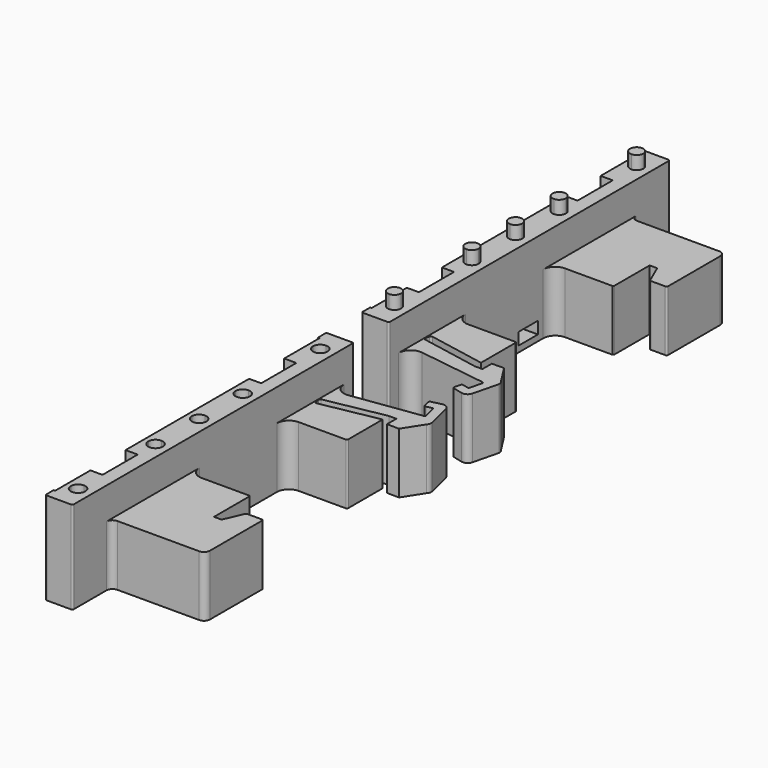
from build123d import *

# Parameters (mm, degrees)
F0_W      = 0.25
F0_H      = 7.25
F0_W_2    = 2
F0_H_2    = 25.5
F1_DEPTH  = 3.5
F2_W      = 4
F2_H      = 2
F3_DEPTH  = 4.5
F5_DEPTH  = 6.5
F7_DEPTH  = 5.25
F9_ANGLE  = 180
F13_DEPTH = 2.4
F14_DEPTH = 2.2


# Not quite as in the source:
# - a feature names something its author has since deleted; it is built from what else it names


with BuildPart() as f1:
    # F0 (on Top) → F1 (new body)
    with BuildSketch(Plane.XY):
        with BuildLine():
            Line((-24.9246123582, 55.1439750494), (-24.9246123582, 35.9745444804))
            ThreePointArc((-24.9246123582, 35.9745444804), (-24.3388259206, 37.3887580428), (-22.9246123582, 37.9745444804))
            Line((-22.9246123582, 37.9745444804), (-15.1132449657, 37.9745444804))
            ThreePointArc((-15.1132449657, 37.9745444804), (-14.974931029, 38.0663469276), (-14.9246123582, 38.2245444804))
            Line((-14.9246123582, 38.2245444804), (-14.9246123582, 45.4523755611))
            Line((-14.9246123582, 45.4523755611), (-13.6746123582, 45.4523755611))
            Line((-13.6746123582, 45.4523755611), (-12.3013395786, 42.2942820054))
            ThreePointArc((-12.3013395786, 42.2942820054), (-12.2091477453, 42.1849017835), (-12.0720770719, 42.1439750494))
            Line((-12.0720770719, 42.1439750494), (-9.7359797508, 42.1439750494))
            ThreePointArc((-9.7359797508, 42.1439750494), (-9.5179749824, 42.1913560505), (-9.4246123582, 42.3939750494))
            Line((-9.4246123582, 42.3939750494), (-9.4246123582, 53.1439750494))
            ThreePointArc((-9.4246123582, 53.1439750494), (-9.717505577, 53.8510818306), (-10.4246123582, 54.1439750494))
            Line((-10.4246123582, 54.1439750494), (-23.9246123582, 54.1439750494))
            ThreePointArc((-23.9246123582, 54.1439750494), (-24.6317191394, 54.4368682682), (-24.9246123582, 55.1439750494))
        make_face()
        with Locations((-29.2996123582, 16.7689750494)):
            Rectangle(F0_W, F0_H)
        with Locations((-29.2996123582, 49.5189750494)):
            Rectangle(F0_W, F0_H)
        with Locations((-29.2996123582, 56.7689750494)):
            Rectangle(F0_W, F0_H)
        with BuildLine():
            Line((-29.4246123582, 5.8939750494), (-29.4246123582, 4.3939750494))
            ThreePointArc((-29.4246123582, 4.3939750494), (-29.3513890535, 4.2171983541), (-29.1746123582, 4.1439750494))
            Line((-29.1746123582, 4.1439750494), (-25.2605436295, 4.1439750494))
            ThreePointArc((-25.2605436295, 4.1439750494), (-25.0248826881, 4.1780111688), (-24.9246123582, 4.3939750494))
            Line((-24.9246123582, 4.3939750494), (-24.9246123582, 6.1439750494))
            Line((-24.9246123582, 6.1439750494), (-24.9246123582, 19.9745444804))
            Line((-24.9246123582, 19.9745444804), (-24.9246123582, 35.9745444804))
            Line((-24.9246123582, 35.9745444804), (-24.9246123582, 55.1439750494))
            Line((-24.9246123582, 55.1439750494), (-24.9246123582, 61.8939750494))
            ThreePointArc((-24.9246123582, 61.8939750494), (-24.9978356629, 62.0707517447), (-25.1746123582, 62.1439750494))
            Line((-25.1746123582, 62.1439750494), (-29.1746123582, 62.1439750494))
            ThreePointArc((-29.1746123582, 62.1439750494), (-29.3513890535, 62.0707517447), (-29.4246123582, 61.8939750494))
            Line((-29.4246123582, 61.8939750494), (-29.4246123582, 60.3939750494))
            Line((-29.4246123582, 60.3939750494), (-29.1746123582, 60.3939750494))
            Line((-29.1746123582, 60.3939750494), (-29.1746123582, 53.1439750494))
            Line((-29.1746123582, 53.1439750494), (-27.1746123582, 53.1439750494))
            Line((-27.1746123582, 53.1439750494), (-27.1746123582, 45.8939750494))
            Line((-27.1746123582, 45.8939750494), (-29.1746123582, 45.8939750494))
            Line((-29.1746123582, 45.8939750494), (-29.1746123582, 20.3939750494))
            Line((-29.1746123582, 20.3939750494), (-27.1746123582, 20.3939750494))
            Line((-27.1746123582, 20.3939750494), (-27.1746123582, 13.1439750494))
            Line((-27.1746123582, 13.1439750494), (-29.1746123582, 13.1439750494))
            Line((-29.1746123582, 13.1439750494), (-29.1746123582, 5.8939750494))
            Line((-29.1746123582, 5.8939750494), (-29.4246123582, 5.8939750494))
        make_face()
        with BuildLine():
            Line((-24.9246123582, 19.9745444804), (-24.9246123582, 6.1439750494))
            ThreePointArc((-24.9246123582, 6.1439750494), (-24.2369140639, 7.6532345477), (-22.646748125, 8.1245788633))
            Line((-22.646748125, 8.1245788633), (-11.4220707577, 6.5498387017))
            ThreePointArc((-11.4220707577, 6.5498387017), (-11.2496628343, 6.442236886), (-11.2141424112, 6.2421345563))
            Line((-11.2141424112, 6.2421345563), (-11.6886017489, 4.3273581574))
            ThreePointArc((-11.6886017489, 4.3273581574), (-11.8021930096, 4.1733819325), (-11.9913917931, 4.1448254504))
            Line((-11.9913917931, 4.1448254504), (-12.8324628729, 4.3532330889))
            ThreePointArc((-12.8324628729, 4.3532330889), (-13.0216616564, 4.3246766068), (-13.1352529171, 4.1707003819))
            Line((-13.1352529171, 4.1707003819), (-13.3757675915, 3.2000548794))
            ThreePointArc((-13.3757675915, 3.2000548794), (-13.3472111095, 3.0108560959), (-13.1932348845, 2.8972648352))
            Line((-13.1932348845, 2.8972648352), (-11.6241796779, 2.508471191))
            ThreePointArc((-11.6241796779, 2.508471191), (-10.8673845438, 2.6226971192), (-10.413019501, 3.238602019))
            Line((-10.413019501, 3.238602019), (-9.3807168548, 7.4046676578))
            ThreePointArc((-9.3807168548, 7.4046676578), (-9.4341945556, 7.8242067251), (-9.6563138888, 8.1841176797))
            Line((-9.6563138888, 8.1841176797), (-11.6748774623, 11.3390995254))
            Line((-11.6748774623, 11.3390995254), (-13.6746123582, 11.3065365708))
            Line((-13.6746123582, 11.3065365708), (-13.6746123582, 9.3696715602))
            Line((-13.6746123582, 9.3696715602), (-14.9246123582, 9.3696715602))
            Line((-14.9246123582, 9.3696715602), (-24.6212489559, 11.1983114075))
            ThreePointArc((-24.6212489559, 11.1983114075), (-24.7813939938, 11.3030263501), (-24.82058899, 11.4903106383))
            Line((-24.82058899, 11.4903106383), (-24.6816001949, 12.2273195357))
            ThreePointArc((-24.6816001949, 12.2273195357), (-24.5768852523, 12.3874645735), (-24.389600964, 12.4266595698))
            Line((-24.389600964, 12.4266595698), (-14.9246123582, 10.6417050504))
            Line((-14.9246123582, 10.6417050504), (-14.9246123582, 17.7245444804))
            ThreePointArc((-14.9246123582, 17.7245444804), (-14.974931029, 17.8827420333), (-15.1132449657, 17.9745444804))
            Line((-15.1132449657, 17.9745444804), (-22.9246123582, 17.9745444804))
            ThreePointArc((-22.9246123582, 17.9745444804), (-24.3388259206, 18.5603309181), (-24.9246123582, 19.9745444804))
        make_face()
        with Locations((-29.2996123582, 9.5189750494)):
            Rectangle(F0_W, F0_H)
        with Locations((-28.1746123582, 16.7689750494)):
            Rectangle(F0_W_2, F0_H)
        with Locations((-28.1746123582, 49.5189750494)):
            Rectangle(F0_W_2, F0_H)
        with Locations((-29.2996123582, 33.1439750494)):
            Rectangle(F0_W, F0_H_2)
    extrude(amount=F1_DEPTH)

    # F2 (on face) → F3 (cut)
    with BuildSketch(Plane(origin=(-29.4246123582, 0, 0), x_dir=(0, -1, 0), z_dir=(-1, 0, 0))):
        with Locations((-32.8939750494, 2)):
            Rectangle(F2_W, F2_H)
    extrude(amount=-F3_DEPTH, mode=Mode.SUBTRACT)

    # F4 (on face) → F5 (join)
    with BuildSketch(Plane.XY.offset(3.5)):
        with BuildLine():
            Line((-29.1746123582, 13.1439750494), (-29.1746123582, 5.8939750494))
            Line((-29.1746123582, 5.8939750494), (-29.4246123582, 5.8939750494))
            Line((-29.4246123582, 5.8939750494), (-29.4246123582, 4.3939750494))
            ThreePointArc((-29.4246123582, 4.3939750494), (-29.3513890535, 4.2171983541), (-29.1746123582, 4.1439750494))
            Line((-29.1746123582, 4.1439750494), (-25.2605436295, 4.1439750494))
            ThreePointArc((-25.2605436295, 4.1439750494), (-25.0248826881, 4.1780111688), (-24.9246123582, 4.3939750494))
            Line((-24.9246123582, 4.3939750494), (-24.9246123582, 6.1439750494))
            ThreePointArc((-24.9246123582, 6.1439750494), (-24.2369140639, 7.6532345477), (-22.646748125, 8.1245788633))
            Line((-22.646748125, 8.1245788633), (-11.4220707577, 6.5498387017))
            ThreePointArc((-11.4220707577, 6.5498387017), (-11.2496628343, 6.442236886), (-11.2141424112, 6.2421345563))
            Line((-11.2141424112, 6.2421345563), (-11.6886017489, 4.3273581574))
            ThreePointArc((-11.6886017489, 4.3273581574), (-11.8021930096, 4.1733819325), (-11.9913917931, 4.1448254504))
            Line((-11.9913917931, 4.1448254504), (-12.8324628729, 4.3532330889))
            ThreePointArc((-12.8324628729, 4.3532330889), (-13.0216616564, 4.3246766068), (-13.1352529171, 4.1707003819))
            Line((-13.1352529171, 4.1707003819), (-13.3757675915, 3.2000548794))
            ThreePointArc((-13.3757675915, 3.2000548794), (-13.3472111095, 3.0108560959), (-13.1932348845, 2.8972648352))
            Line((-13.1932348845, 2.8972648352), (-11.6241796779, 2.508471191))
            ThreePointArc((-11.6241796779, 2.508471191), (-10.8673845438, 2.6226971192), (-10.413019501, 3.238602019))
            Line((-10.413019501, 3.238602019), (-9.3807168548, 7.4046676578))
            ThreePointArc((-9.3807168548, 7.4046676578), (-9.4341945556, 7.8242067251), (-9.6563138888, 8.1841176797))
            Line((-9.6563138888, 8.1841176797), (-11.6748774623, 11.3390995254))
            Line((-11.6748774623, 11.3390995254), (-13.6746123582, 11.3065365708))
            Line((-13.6746123582, 11.3065365708), (-13.6746123582, 9.3696715602))
            Line((-13.6746123582, 9.3696715602), (-14.9246123582, 9.3696715602))
            Line((-14.9246123582, 9.3696715602), (-24.6212489559, 11.1983114075))
            ThreePointArc((-24.6212489559, 11.1983114075), (-24.7813939938, 11.3030263501), (-24.82058899, 11.4903106383))
            Line((-24.82058899, 11.4903106383), (-24.6816001949, 12.2273195357))
            ThreePointArc((-24.6816001949, 12.2273195357), (-24.5768852523, 12.3874645735), (-24.389600964, 12.4266595698))
            Line((-24.389600964, 12.4266595698), (-14.9246123582, 10.6417050504))
            Line((-14.9246123582, 10.6417050504), (-14.9246123582, 17.7245444804))
            ThreePointArc((-14.9246123582, 17.7245444804), (-14.974931029, 17.8827420333), (-15.1132449657, 17.9745444804))
            Line((-15.1132449657, 17.9745444804), (-22.9246123582, 17.9745444804))
            ThreePointArc((-22.9246123582, 17.9745444804), (-24.3388259206, 18.5603309181), (-24.9246123582, 19.9745444804))
            Line((-24.9246123582, 19.9745444804), (-24.9246123582, 35.9745444804))
            ThreePointArc((-24.9246123582, 35.9745444804), (-24.3388259206, 37.3887580428), (-22.9246123582, 37.9745444804))
            Line((-22.9246123582, 37.9745444804), (-15.1132449657, 37.9745444804))
            ThreePointArc((-15.1132449657, 37.9745444804), (-14.974931029, 38.0663469276), (-14.9246123582, 38.2245444804))
            Line((-14.9246123582, 38.2245444804), (-14.9246123582, 45.4523755611))
            Line((-14.9246123582, 45.4523755611), (-13.6746123582, 45.4523755611))
            Line((-13.6746123582, 45.4523755611), (-12.3013395786, 42.2942820054))
            ThreePointArc((-12.3013395786, 42.2942820054), (-12.2091477453, 42.1849017835), (-12.0720770719, 42.1439750494))
            Line((-12.0720770719, 42.1439750494), (-9.7359797508, 42.1439750494))
            ThreePointArc((-9.7359797508, 42.1439750494), (-9.5179749824, 42.1913560505), (-9.4246123582, 42.3939750494))
            Line((-9.4246123582, 42.3939750494), (-9.4246123582, 53.1439750494))
            ThreePointArc((-9.4246123582, 53.1439750494), (-9.717505577, 53.8510818306), (-10.4246123582, 54.1439750494))
            Line((-10.4246123582, 54.1439750494), (-23.9246123582, 54.1439750494))
            ThreePointArc((-23.9246123582, 54.1439750494), (-24.6317191394, 54.4368682682), (-24.9246123582, 55.1439750494))
            Line((-24.9246123582, 55.1439750494), (-24.9246123582, 61.8939750494))
            ThreePointArc((-24.9246123582, 61.8939750494), (-24.9978356629, 62.0707517447), (-25.1746123582, 62.1439750494))
            Line((-25.1746123582, 62.1439750494), (-29.1746123582, 62.1439750494))
            ThreePointArc((-29.1746123582, 62.1439750494), (-29.3513890535, 62.0707517447), (-29.4246123582, 61.8939750494))
            Line((-29.4246123582, 61.8939750494), (-29.4246123582, 60.3939750494))
            Line((-29.4246123582, 60.3939750494), (-29.1746123582, 60.3939750494))
            Line((-29.1746123582, 60.3939750494), (-29.1746123582, 53.1439750494))
            Line((-29.1746123582, 53.1439750494), (-27.1746123582, 53.1439750494))
            Line((-27.1746123582, 53.1439750494), (-27.1746123582, 45.8939750494))
            Line((-27.1746123582, 45.8939750494), (-29.1746123582, 45.8939750494))
            Line((-29.1746123582, 45.8939750494), (-29.1746123582, 20.3939750494))
            Line((-29.1746123582, 20.3939750494), (-27.1746123582, 20.3939750494))
            Line((-27.1746123582, 20.3939750494), (-27.1746123582, 13.1439750494))
            Line((-27.1746123582, 13.1439750494), (-29.1746123582, 13.1439750494))
        make_face()
    extrude(amount=F5_DEPTH)

    # F6 (on face) → F7 (join)
    with BuildSketch(Plane.XY.offset(10)):
        with BuildLine():
            Line((-24.9246123582, 55.1439750494), (-24.9246123582, 61.8939750494))
            ThreePointArc((-24.9246123582, 61.8939750494), (-24.9978356629, 62.0707517447), (-25.1746123582, 62.1439750494))
            Line((-25.1746123582, 62.1439750494), (-29.1746123582, 62.1439750494))
            ThreePointArc((-29.1746123582, 62.1439750494), (-29.3513890535, 62.0707517447), (-29.4246123582, 61.8939750494))
            Line((-29.4246123582, 61.8939750494), (-29.4246123582, 60.3939750494))
            Line((-29.4246123582, 60.3939750494), (-29.1746123582, 60.3939750494))
            Line((-29.1746123582, 60.3939750494), (-29.1746123582, 53.1439750494))
            Line((-29.1746123582, 53.1439750494), (-27.1746123582, 53.1439750494))
            Line((-27.1746123582, 53.1439750494), (-27.1746123582, 45.8939750494))
            Line((-27.1746123582, 45.8939750494), (-29.1746123582, 45.8939750494))
            Line((-29.1746123582, 45.8939750494), (-29.1746123582, 20.3939750494))
            Line((-29.1746123582, 20.3939750494), (-27.1746123582, 20.3939750494))
            Line((-27.1746123582, 20.3939750494), (-27.1746123582, 13.1439750494))
            Line((-27.1746123582, 13.1439750494), (-29.1746123582, 13.1439750494))
            Line((-29.1746123582, 13.1439750494), (-29.1746123582, 5.8939750494))
            Line((-29.1746123582, 5.8939750494), (-29.4246123582, 5.8939750494))
            Line((-29.4246123582, 5.8939750494), (-29.4246123582, 4.3939750494))
            ThreePointArc((-29.4246123582, 4.3939750494), (-29.3513890535, 4.2171983541), (-29.1746123582, 4.1439750494))
            Line((-29.1746123582, 4.1439750494), (-25.2605436295, 4.1439750494))
            ThreePointArc((-25.2605436295, 4.1439750494), (-25.0248826881, 4.1780111688), (-24.9246123582, 4.3939750494))
            Line((-24.9246123582, 4.3939750494), (-24.9246123582, 6.1439750494))
            Line((-24.9246123582, 6.1439750494), (-24.9246123582, 19.9745444804))
            Line((-24.9246123582, 19.9745444804), (-24.9246123582, 35.9745444804))
            Line((-24.9246123582, 35.9745444804), (-24.9246123582, 55.1439750494))
        make_face()
    extrude(amount=F7_DEPTH)


with BuildPart() as f8_1:
    # F8: instance of F1
    add(f1.part.mirror(Plane(origin=(-26.9091228203, 33.1433301919, 15.25), x_dir=(1, 0, 0), z_dir=(0, 0, 1))))


with BuildPart() as f8_1_1:
    # F9: moved
    add(f8_1.part.rotate(Axis((-27.1746123582, 62.1439750494, 15.25), (1, 0, 0)), F9_ANGLE))


with BuildPart() as f8_1_2:
    # F10: moved
    add(f8_1_1.part.moved(Location((0, -123.3, 0))))

    # F12 (on face) → F13 (cut)
    with BuildSketch(Plane.XY.offset(15.25)):
        with BuildLine():
            Line((-27.2175779939, -58.3560249506), (-27.2175779939, -57.1560249506))
            Line((-27.2175779939, -57.1560249506), (-28.4175779939, -57.1560249506))
            ThreePointArc((-28.4175779939, -57.1560249506), (-28.0661061313, -58.004553088), (-27.2175779939, -58.3560249506))
        make_face()
        with BuildLine():
            Line((-27.2175779939, -57.1560249506), (-27.2175779939, -55.9560249506))
            ThreePointArc((-27.2175779939, -55.9560249506), (-28.0661061313, -56.3074968132), (-28.4175779939, -57.1560249506))
            Line((-28.4175779939, -57.1560249506), (-27.2175779939, -57.1560249506))
        make_face()
        with BuildLine():
            ThreePointArc((-26.0175779939, -57.1560249506), (-26.3690498564, -56.3074968132), (-27.2175779939, -55.9560249506))
            Line((-27.2175779939, -55.9560249506), (-27.2175779939, -57.1560249506))
            Line((-27.2175779939, -57.1560249506), (-26.0175779939, -57.1560249506))
        make_face()
        with BuildLine():
            Line((-26.0175779939, -57.1560249506), (-27.2175779939, -57.1560249506))
            Line((-27.2175779939, -57.1560249506), (-27.2175779939, -58.3560249506))
            ThreePointArc((-27.2175779939, -58.3560249506), (-26.3690498564, -58.004553088), (-26.0175779939, -57.1560249506))
        make_face()
        with BuildLine():
            Line((-27.2175779939, -33.3560249506), (-27.2175779939, -32.1560249506))
            Line((-27.2175779939, -32.1560249506), (-28.4175779939, -32.1560249506))
            ThreePointArc((-28.4175779939, -32.1560249506), (-28.0661061313, -33.004553088), (-27.2175779939, -33.3560249506))
        make_face()
        with BuildLine():
            Line((-27.2175779939, -32.1560249506), (-27.2175779939, -30.9560249506))
            ThreePointArc((-27.2175779939, -30.9560249506), (-28.0661061313, -31.3074968132), (-28.4175779939, -32.1560249506))
            Line((-28.4175779939, -32.1560249506), (-27.2175779939, -32.1560249506))
        make_face()
        with BuildLine():
            ThreePointArc((-26.0175779939, -32.1560249506), (-26.3690498564, -31.3074968132), (-27.2175779939, -30.9560249506))
            Line((-27.2175779939, -30.9560249506), (-27.2175779939, -32.1560249506))
            Line((-27.2175779939, -32.1560249506), (-26.0175779939, -32.1560249506))
        make_face()
        with BuildLine():
            Line((-26.0175779939, -32.1560249506), (-27.2175779939, -32.1560249506))
            Line((-27.2175779939, -32.1560249506), (-27.2175779939, -33.3560249506))
            ThreePointArc((-27.2175779939, -33.3560249506), (-26.3690498564, -33.004553088), (-26.0175779939, -32.1560249506))
        make_face()
        with BuildLine():
            Line((-27.2175779939, -8.3560249506), (-27.2175779939, -7.1560249506))
            Line((-27.2175779939, -7.1560249506), (-28.4175779939, -7.1560249506))
            ThreePointArc((-28.4175779939, -7.1560249506), (-28.0661061313, -8.004553088), (-27.2175779939, -8.3560249506))
        make_face()
        with BuildLine():
            Line((-27.2175779939, -7.1560249506), (-27.2175779939, -5.9560249506))
            ThreePointArc((-27.2175779939, -5.9560249506), (-28.0661061313, -6.3074968132), (-28.4175779939, -7.1560249506))
            Line((-28.4175779939, -7.1560249506), (-27.2175779939, -7.1560249506))
        make_face()
        with BuildLine():
            ThreePointArc((-26.0175779939, -7.1560249506), (-26.3690498564, -6.3074968132), (-27.2175779939, -5.9560249506))
            Line((-27.2175779939, -5.9560249506), (-27.2175779939, -7.1560249506))
            Line((-27.2175779939, -7.1560249506), (-26.0175779939, -7.1560249506))
        make_face()
        with BuildLine():
            Line((-26.0175779939, -7.1560249506), (-27.2175779939, -7.1560249506))
            Line((-27.2175779939, -7.1560249506), (-27.2175779939, -8.3560249506))
            ThreePointArc((-27.2175779939, -8.3560249506), (-26.3690498564, -8.004553088), (-26.0175779939, -7.1560249506))
        make_face()
        with BuildLine():
            Line((-27.2175779939, -41.1560249506), (-27.2175779939, -39.9560249506))
            ThreePointArc((-27.2175779939, -39.9560249506), (-28.0661061313, -40.3074968132), (-28.4175779939, -41.1560249506))
            Line((-28.4175779939, -41.1560249506), (-27.2175779939, -41.1560249506))
        make_face()
        with BuildLine():
            Line((-27.2175779939, -42.3560249506), (-27.2175779939, -41.1560249506))
            Line((-27.2175779939, -41.1560249506), (-28.4175779939, -41.1560249506))
            ThreePointArc((-28.4175779939, -41.1560249506), (-28.0661061313, -42.004553088), (-27.2175779939, -42.3560249506))
        make_face()
        with BuildLine():
            Line((-26.0175779939, -41.1560249506), (-27.2175779939, -41.1560249506))
            Line((-27.2175779939, -41.1560249506), (-27.2175779939, -42.3560249506))
            ThreePointArc((-27.2175779939, -42.3560249506), (-26.3690498564, -42.004553088), (-26.0175779939, -41.1560249506))
        make_face()
        with BuildLine():
            ThreePointArc((-26.0175779939, -41.1560249506), (-26.3690498564, -40.3074968132), (-27.2175779939, -39.9560249506))
            Line((-27.2175779939, -39.9560249506), (-27.2175779939, -41.1560249506))
            Line((-27.2175779939, -41.1560249506), (-26.0175779939, -41.1560249506))
        make_face()
        with BuildLine():
            Line((-26.0175779939, -23.1560249506), (-27.2175779939, -23.1560249506))
            Line((-27.2175779939, -23.1560249506), (-27.2175779939, -24.3560249506))
            ThreePointArc((-27.2175779939, -24.3560249506), (-26.3690498564, -24.004553088), (-26.0175779939, -23.1560249506))
        make_face()
        with BuildLine():
            ThreePointArc((-26.0175779939, -23.1560249506), (-26.3690498564, -22.3074968132), (-27.2175779939, -21.9560249506))
            Line((-27.2175779939, -21.9560249506), (-27.2175779939, -23.1560249506))
            Line((-27.2175779939, -23.1560249506), (-26.0175779939, -23.1560249506))
        make_face()
        with BuildLine():
            Line((-27.2175779939, -23.1560249506), (-27.2175779939, -21.9560249506))
            ThreePointArc((-27.2175779939, -21.9560249506), (-28.0661061313, -22.3074968132), (-28.4175779939, -23.1560249506))
            Line((-28.4175779939, -23.1560249506), (-27.2175779939, -23.1560249506))
        make_face()
        with BuildLine():
            Line((-27.2175779939, -24.3560249506), (-27.2175779939, -23.1560249506))
            Line((-27.2175779939, -23.1560249506), (-28.4175779939, -23.1560249506))
            ThreePointArc((-28.4175779939, -23.1560249506), (-28.0661061313, -24.004553088), (-27.2175779939, -24.3560249506))
        make_face()
    extrude(amount=-F13_DEPTH, mode=Mode.SUBTRACT)


with BuildPart() as f1_1:
    add(f1.part)

    # F11 (on face) → F14 (join)
    with BuildSketch(Plane.XY.offset(15.25)):
        with BuildLine():
            ThreePointArc((-28.3175779939, 33.1439750494), (-27.9953954532, 32.3661575901), (-27.2175779939, 32.0439750494))
            Line((-27.2175779939, 32.0439750494), (-27.2175779939, 33.1439750494))
            Line((-27.2175779939, 33.1439750494), (-28.3175779939, 33.1439750494))
        make_face()
        with BuildLine():
            Line((-28.3175779939, 33.1439750494), (-27.2175779939, 33.1439750494))
            Line((-27.2175779939, 33.1439750494), (-27.2175779939, 34.2439750494))
            ThreePointArc((-27.2175779939, 34.2439750494), (-27.9953954532, 33.9217925087), (-28.3175779939, 33.1439750494))
        make_face()
        with BuildLine():
            Line((-27.2175779939, 33.1439750494), (-26.1175779939, 33.1439750494))
            ThreePointArc((-26.1175779939, 33.1439750494), (-26.4397605346, 33.9217925087), (-27.2175779939, 34.2439750494))
            Line((-27.2175779939, 34.2439750494), (-27.2175779939, 33.1439750494))
        make_face()
        with BuildLine():
            ThreePointArc((-27.2175779939, 32.0439750494), (-26.4397605346, 32.3661575901), (-26.1175779939, 33.1439750494))
            Line((-26.1175779939, 33.1439750494), (-27.2175779939, 33.1439750494))
            Line((-27.2175779939, 33.1439750494), (-27.2175779939, 32.0439750494))
        make_face()
        with BuildLine():
            Line((-28.3175779939, 58.1439750494), (-27.2175779939, 58.1439750494))
            Line((-27.2175779939, 58.1439750494), (-27.2175779939, 59.2439750494))
            ThreePointArc((-27.2175779939, 59.2439750494), (-27.9953954532, 58.9217925087), (-28.3175779939, 58.1439750494))
        make_face()
        with BuildLine():
            Line((-27.2175779939, 57.0439750494), (-27.2175779939, 58.1439750494))
            Line((-27.2175779939, 58.1439750494), (-28.3175779939, 58.1439750494))
            ThreePointArc((-28.3175779939, 58.1439750494), (-27.9953954532, 57.3661575901), (-27.2175779939, 57.0439750494))
        make_face()
        with BuildLine():
            ThreePointArc((-27.2175779939, 57.0439750494), (-26.4397605346, 57.3661575901), (-26.1175779939, 58.1439750494))
            Line((-26.1175779939, 58.1439750494), (-27.2175779939, 58.1439750494))
            Line((-27.2175779939, 58.1439750494), (-27.2175779939, 57.0439750494))
        make_face()
        with BuildLine():
            Line((-27.2175779939, 58.1439750494), (-26.1175779939, 58.1439750494))
            ThreePointArc((-26.1175779939, 58.1439750494), (-26.4397605346, 58.9217925087), (-27.2175779939, 59.2439750494))
            Line((-27.2175779939, 59.2439750494), (-27.2175779939, 58.1439750494))
        make_face()
        with BuildLine():
            Line((-28.3175779939, 8.1439750494), (-27.2175779939, 8.1439750494))
            Line((-27.2175779939, 8.1439750494), (-27.2175779939, 9.2439750494))
            ThreePointArc((-27.2175779939, 9.2439750494), (-27.9953954532, 8.9217925087), (-28.3175779939, 8.1439750494))
        make_face()
        with BuildLine():
            ThreePointArc((-28.3175779939, 8.1439750494), (-27.9953954532, 7.3661575901), (-27.2175779939, 7.0439750494))
            Line((-27.2175779939, 7.0439750494), (-27.2175779939, 8.1439750494))
            Line((-27.2175779939, 8.1439750494), (-28.3175779939, 8.1439750494))
        make_face()
        with BuildLine():
            Line((-27.2175779939, 8.1439750494), (-27.2175779939, 7.0439750494))
            ThreePointArc((-27.2175779939, 7.0439750494), (-26.4397605346, 7.3661575901), (-26.1175779939, 8.1439750494))
            Line((-26.1175779939, 8.1439750494), (-27.2175779939, 8.1439750494))
        make_face()
        with BuildLine():
            Line((-27.2175779939, 9.2439750494), (-27.2175779939, 8.1439750494))
            Line((-27.2175779939, 8.1439750494), (-26.1175779939, 8.1439750494))
            ThreePointArc((-26.1175779939, 8.1439750494), (-26.4397605346, 8.9217925087), (-27.2175779939, 9.2439750494))
        make_face()
        with BuildLine():
            Line((-28.3175779939, 24.1439750494), (-27.2175779939, 24.1439750494))
            Line((-27.2175779939, 24.1439750494), (-27.2175779939, 25.2439750494))
            ThreePointArc((-27.2175779939, 25.2439750494), (-27.9953954532, 24.9217925087), (-28.3175779939, 24.1439750494))
        make_face()
        with BuildLine():
            ThreePointArc((-28.3175779939, 24.1439750494), (-27.9953954532, 23.3661575901), (-27.2175779939, 23.0439750494))
            Line((-27.2175779939, 23.0439750494), (-27.2175779939, 24.1439750494))
            Line((-27.2175779939, 24.1439750494), (-28.3175779939, 24.1439750494))
        make_face()
        with BuildLine():
            ThreePointArc((-27.2175779939, 23.0439750494), (-26.4397605346, 23.3661575901), (-26.1175779939, 24.1439750494))
            Line((-26.1175779939, 24.1439750494), (-27.2175779939, 24.1439750494))
            Line((-27.2175779939, 24.1439750494), (-27.2175779939, 23.0439750494))
        make_face()
        with BuildLine():
            Line((-27.2175779939, 24.1439750494), (-26.1175779939, 24.1439750494))
            ThreePointArc((-26.1175779939, 24.1439750494), (-26.4397605346, 24.9217925087), (-27.2175779939, 25.2439750494))
            Line((-27.2175779939, 25.2439750494), (-27.2175779939, 24.1439750494))
        make_face()
        with BuildLine():
            Line((-28.3175779939, 42.1439750494), (-27.2175779939, 42.1439750494))
            Line((-27.2175779939, 42.1439750494), (-27.2175779939, 43.2439750494))
            ThreePointArc((-27.2175779939, 43.2439750494), (-27.9953954532, 42.9217925087), (-28.3175779939, 42.1439750494))
        make_face()
        with BuildLine():
            Line((-27.2175779939, 42.1439750494), (-26.1175779939, 42.1439750494))
            ThreePointArc((-26.1175779939, 42.1439750494), (-26.4397605346, 42.9217925087), (-27.2175779939, 43.2439750494))
            Line((-27.2175779939, 43.2439750494), (-27.2175779939, 42.1439750494))
        make_face()
        with BuildLine():
            ThreePointArc((-27.2175779939, 41.0439750494), (-26.4397605346, 41.3661575901), (-26.1175779939, 42.1439750494))
            Line((-26.1175779939, 42.1439750494), (-27.2175779939, 42.1439750494))
            Line((-27.2175779939, 42.1439750494), (-27.2175779939, 41.0439750494))
        make_face()
        with BuildLine():
            ThreePointArc((-28.3175779939, 42.1439750494), (-27.9953954532, 41.3661575901), (-27.2175779939, 41.0439750494))
            Line((-27.2175779939, 41.0439750494), (-27.2175779939, 42.1439750494))
            Line((-27.2175779939, 42.1439750494), (-28.3175779939, 42.1439750494))
        make_face()
    extrude(amount=F14_DEPTH)


solid = Compound([f8_1_2.part, f1_1.part])
